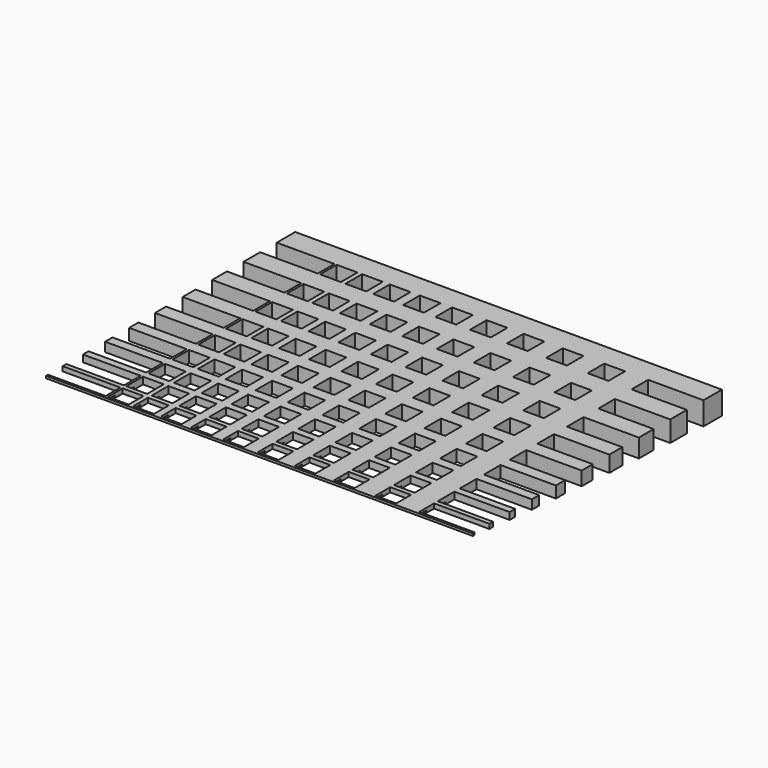
from build123d import *

# Parameters (mm, degrees)
F0_W         = 185
F0_H         = 10
F2_DEPTH     = 10
F0_H_2       = 1
F0_H_3       = 9
F0_H_4       = 8
F0_H_5       = 7
F0_H_6       = 6
F0_H_7       = 5
F0_H_8       = 4
F0_H_9       = 3
F0_H_10      = 2
F1_W         = 10
F1_H         = 135
F1_W_2       = 9
F1_W_3       = 8
F1_W_4       = 7
F1_W_5       = 6
F1_W_6       = 5
F1_W_7       = 4
F1_W_8       = 3
F1_W_9       = 2
F1_W_10      = 1
F3_DEPTH     = 10
F6_DEPTH     = 199.7170002589
F7_TEXT_SIZE = 6.9444444444
F8_DEPTH     = 1


# Not quite as in the source:
# - Text() gives the source's letters only with a copy of the font that has no kerning and outlines rounded to 1/6400 em; it was checked with that copy


with BuildPart() as f2:
    # F0 (on Top) → F2 (new body)
    with BuildSketch(Plane.XY):
        with Locations((-7.2160002589, 71)):
            Rectangle(F0_W, F0_H)
    extrude(amount=F2_DEPTH)



with BuildPart() as f2b:
    # F0 (on Top) → F2, piece 2 (new body)
    with BuildSketch(Plane.XY):
        with Locations((-7.2160002589, -58.5)):
            Rectangle(F0_W, F0_H_2)
    extrude(amount=F2_DEPTH)


with BuildPart() as f2c:
    # F0 (on Top) → F2, piece 3 (new body)
    with BuildSketch(Plane.XY):
        with Locations((-7.2160002589, 52.5)):
            Rectangle(F0_W, F0_H_3)
    extrude(amount=F2_DEPTH)


with BuildPart() as f2d:
    # F0 (on Top) → F2, piece 4 (new body)
    with BuildSketch(Plane.XY):
        with Locations((-7.2160002589, 35)):
            Rectangle(F0_W, F0_H_4)
    extrude(amount=F2_DEPTH)


with BuildPart() as f2e:
    # F0 (on Top) → F2, piece 5 (new body)
    with BuildSketch(Plane.XY):
        with Locations((-7.2160002589, 18.5)):
            Rectangle(F0_W, F0_H_5)
    extrude(amount=F2_DEPTH)


with BuildPart() as f2f:
    # F0 (on Top) → F2, piece 6 (new body)
    with BuildSketch(Plane.XY):
        with Locations((-7.2160002589, 3)):
            Rectangle(F0_W, F0_H_6)
    extrude(amount=F2_DEPTH)


with BuildPart() as f2g:
    # F0 (on Top) → F2, piece 7 (new body)
    with BuildSketch(Plane.XY):
        with Locations((-7.2160002589, -11.5)):
            Rectangle(F0_W, F0_H_7)
    extrude(amount=F2_DEPTH)


with BuildPart() as f2h:
    # F0 (on Top) → F2, piece 8 (new body)
    with BuildSketch(Plane.XY):
        with Locations((-7.2160002589, -25)):
            Rectangle(F0_W, F0_H_8)
    extrude(amount=F2_DEPTH)


with BuildPart() as f2i:
    # F0 (on Top) → F2, piece 9 (new body)
    with BuildSketch(Plane.XY):
        with Locations((-7.2160002589, -37.5)):
            Rectangle(F0_W, F0_H_9)
    extrude(amount=F2_DEPTH)


with BuildPart() as f2j:
    # F0 (on Top) → F2, piece 10 (new body)
    with BuildSketch(Plane.XY):
        with Locations((-7.2160002589, -49)):
            Rectangle(F0_W, F0_H_10)
    extrude(amount=F2_DEPTH)


with BuildPart() as f2_1:
    add(f2.part)

    add(f2b.part)  # F3 merges F2b

    add(f2c.part)  # F3 merges F2c

    add(f2d.part)  # F3 merges F2d

    add(f2e.part)  # F3 merges F2e

    add(f2f.part)  # F3 merges F2f

    add(f2g.part)  # F3 merges F2g

    add(f2h.part)  # F3 merges F2h

    add(f2i.part)  # F3 merges F2i

    add(f2j.part)  # F3 merges F2j
    # F1 (on Top) → F3 (join)
    with BuildSketch(Plane.XY):
        with Locations((56.2839997411, 8.5)):
            Rectangle(F1_W, F1_H)
        with Locations((37.7839997411, 8.5)):
            Rectangle(F1_W_2, F1_H)
        with Locations((20.2839997411, 8.5)):
            Rectangle(F1_W_3, F1_H)
        with Locations((3.7839997411, 8.5)):
            Rectangle(F1_W_4, F1_H)
        with Locations((-11.7160002589, 8.5)):
            Rectangle(F1_W_5, F1_H)
        with Locations((-26.2160002589, 8.5)):
            Rectangle(F1_W_6, F1_H)
        with Locations((-39.7160002589, 8.5)):
            Rectangle(F1_W_7, F1_H)
        with Locations((-52.2160002589, 8.5)):
            Rectangle(F1_W_8, F1_H)
        with Locations((-63.7160002589, 8.5)):
            Rectangle(F1_W_9, F1_H)
        with Locations((-74.2160002589, 8.5)):
            Rectangle(F1_W_10, F1_H)
    extrude(amount=F3_DEPTH)

    # F5 (on offset) → F6 (cut, through all)
    with BuildSketch(Plane.YZ.offset(100)):
        Polygon((-63.8573838881, 0), (61.4425465465, 0), (61.4425465465, 1), (43.861284852, 1), (43.861284852, 2), (26.5515675498, 2), (26.5515675498, 3), (10.4473830216, 3), (10.4473830216, 4), (-4.7310536771, 4), (-4.7310536771, 5), (-18.4628582929, 5), (-18.4628582929, 6), (-31.4343999211, 6), (-31.4343999211, 7), (-43.8079816057, 7), (-43.8079816057, 8), (-54.1132406702, 8), (-54.1132406702, 9), (-63.8573838881, 9), align=None)
    extrude(amount=-F6_DEPTH, mode=Mode.SUBTRACT)

    # F7 (on face) → F8 (join)
    with BuildSketch(Plane(origin=(0, 0, 0), x_dir=(1, 0, 0), z_dir=(0, 0, -1))):
        with Locations((-16.0356840535, -73.6508091357)):
            Text('C', F7_TEXT_SIZE, font='Open Sans', font_style=FontStyle.BOLD, text_align=(TextAlign.LEFT, TextAlign.BOTTOM))
    extrude(amount=F8_DEPTH)


solid = f2_1.part
